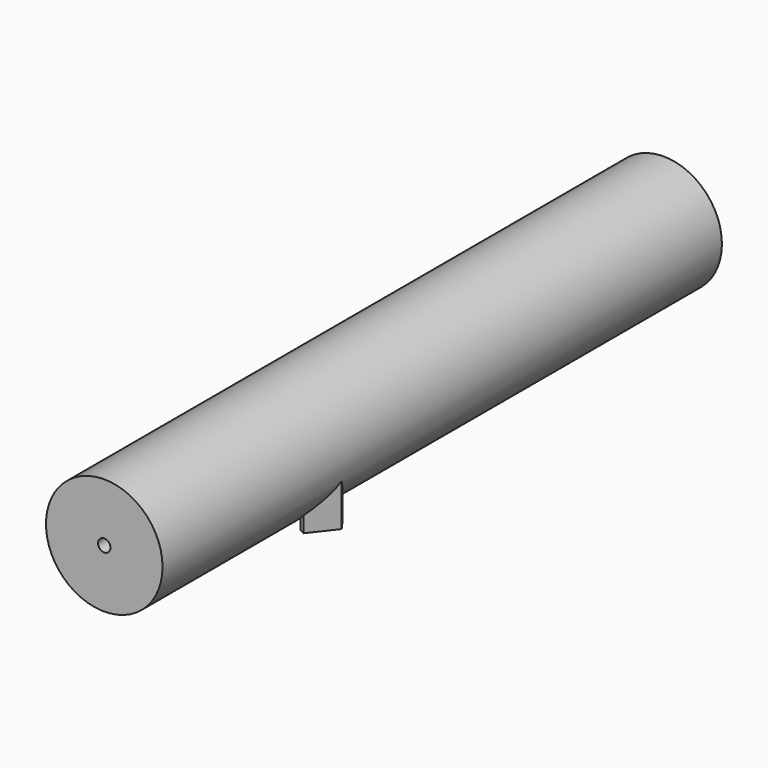
from build123d import *

# Parameters (mm, degrees)
F0_R         = 15
F0_R_2       = 12
F1_DEPTH     = 180
F2_DEPTH     = 160
F5_DEPTH     = 20
F6_DEPTH     = 18
F7_DEPTH     = 0.5
F8_DEPTH     = 160
F9_T1_DEPTH  = 33.1189779758
F10_T1_DEPTH = 33.1189779758
F11_R        = 1.6
F12_DEPTH    = 20


# Not quite as in the source:
# - a fillet or chamfer that OpenCascade refuses, or shapes differently, is made with other operations: its cross-section is extruded or revolved along the edge and cut away or added


with BuildPart() as f1:
    # F0 (on Front) → F1 (new body)
    with BuildSketch(Plane.XZ):
        Circle(F0_R)
        Circle(F0_R_2, mode=Mode.SUBTRACT)
        Circle(F0_R_2)
    extrude(amount=F1_DEPTH)

    # F0 (on Front) → F2 (cut)
    with BuildSketch(Plane.XZ):
        Circle(F0_R_2)
    extrude(amount=F2_DEPTH, mode=Mode.SUBTRACT)

    # F4 (on offset) → F5 (cut)
    with BuildSketch(Plane.XY.offset(-15)):
        with BuildLine():
            ThreePointArc((10.5, -117.0782160674), (5.5711218584, -114.3097131563), (0, -113.35))
            Line((0, -113.35), (0, -130))
            Line((0, -130), (7, -130))
            Line((7, -130), (10.5, -130))
            Line((10.5, -130), (10.5, -117.0782160674))
        make_face()
        with BuildLine():
            Line((0, -130), (0, -113.35))
            ThreePointArc((0, -113.35), (-5.5711218584, -114.3097131563), (-10.5, -117.0782160674))
            Line((-10.5, -117.0782160674), (-10.5, -130))
            Line((-10.5, -130), (-7, -130))
            Line((-7, -130), (0, -130))
        make_face()
    extrude(amount=F5_DEPTH, mode=Mode.SUBTRACT)

    # F4 (on offset) → F6 (join)
    with BuildSketch(Plane.XY.offset(-15)):
        with BuildLine():
            ThreePointArc((14.2855073516, -121.4474109355), (12.5838312774, -119.0972622529), (10.5, -117.0782160674))
            Line((10.5, -117.0782160674), (10.5, -130))
            Line((10.5, -130), (11.29, -130))
            Line((11.29, -130), (14.2855073516, -121.4474109355))
        make_face()
        with BuildLine():
            Line((-10.5, -130), (-10.5, -117.0782160674))
            ThreePointArc((-10.5, -117.0782160674), (-12.5838312774, -119.0972622529), (-14.2855073516, -121.4474109355))
            Line((-14.2855073516, -121.4474109355), (-11.29, -130))
            Line((-11.29, -130), (-10.5, -130))
        make_face()
    extrude(amount=F6_DEPTH)

    # F4 (on offset) → F7 (join)
    with BuildSketch(Plane.XY.offset(-15)):
        with BuildLine():
            Line((-10.5, -130), (-10.5, -117.0782160674))
            ThreePointArc((-10.5, -117.0782160674), (-12.5838312774, -119.0972622529), (-14.2855073516, -121.4474109355))
            Line((-14.2855073516, -121.4474109355), (-11.29, -130))
            Line((-11.29, -130), (-10.5, -130))
        make_face()
        with BuildLine():
            ThreePointArc((14.2855073516, -121.4474109355), (12.5838312774, -119.0972622529), (10.5, -117.0782160674))
            Line((10.5, -117.0782160674), (10.5, -130))
            Line((10.5, -130), (11.29, -130))
            Line((11.29, -130), (14.2855073516, -121.4474109355))
        make_face()
    extrude(amount=-F7_DEPTH)

    # F0 (on Front) → F8 (cut)
    with BuildSketch(Plane.XZ):
        Circle(F0_R_2)
    extrude(amount=F8_DEPTH, mode=Mode.SUBTRACT)

    # F9: chamfer of 3.9 x 2 on 1 edges, made by hand

    # F9_s2 → F9_t1 (cut)
    with BuildSketch(Plane.XZ.offset(106.9796190458)):
        Polygon((10.5, -13.5), (14.4, -15.5), (10.5, -15.5), align=None)
    extrude(amount=F9_T1_DEPTH, mode=Mode.SUBTRACT)

    # F10: chamfer of 2 x 3.9 on 1 edges, made by hand

    # F10_s2 → F10_t1 (cut)
    with BuildSketch(Plane.XZ.offset(106.9796190458)):
        Polygon((-10.5, -13.5), (-14.4, -15.5), (-10.5, -15.5), align=None)
    extrude(amount=F10_T1_DEPTH, mode=Mode.SUBTRACT)

    # F11 (on face) → F12 (cut)
    with BuildSketch(Plane.XZ.offset(180)):
        Circle(F11_R)
    extrude(amount=-F12_DEPTH, mode=Mode.SUBTRACT)


solid = f1.part
